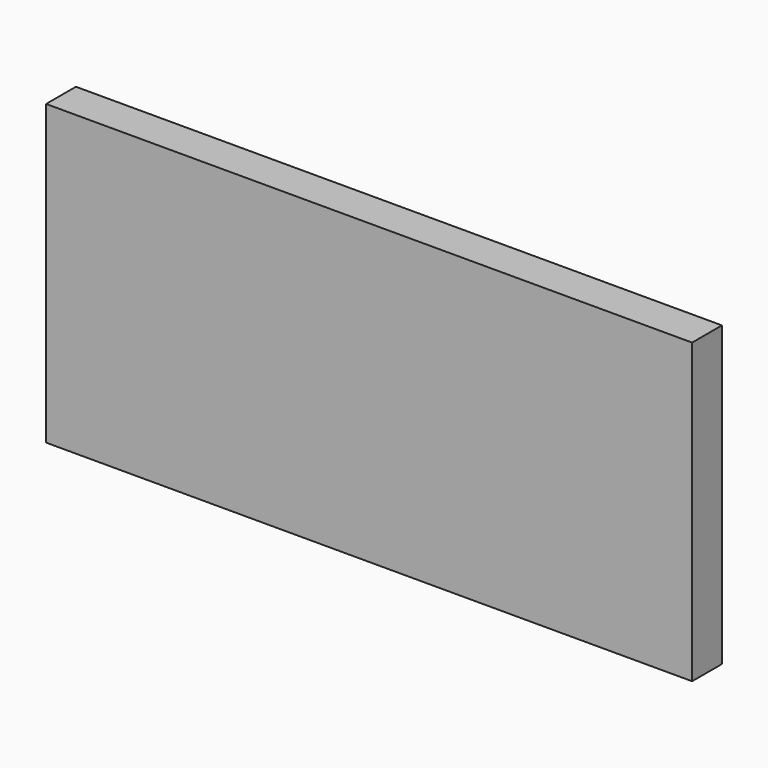
from build123d import *

# Parameters (mm, degrees)
F0_W     = 381
F0_H     = 152.4
F1_DEPTH = 25.4
F3_W     = 330.2
F3_H     = 152.4
F4_DEPTH = 19.05


# Not quite as in the source:
# - a length typed as a fraction of an inch, garbled in the dataset ("3 / 203.2 mm" for 3/8 in), is restored


with BuildPart() as f1:
    # F0 (on Front) → F1 (new body)
    with BuildSketch(Plane.XZ):
        with Locations((-29.8060849309, -110.5314957584)):
            Rectangle(F0_W, F0_H)
    extrude(amount=F1_DEPTH)


with BuildPart() as f4:
    # F3 (on Front) → F4 (new body)
    with BuildSketch(Plane.XZ):
        with Locations((-81.6316027194, -59.3715892611)):
            Rectangle(F3_W, F3_H)
    extrude(amount=F4_DEPTH)


solid = f4.part
